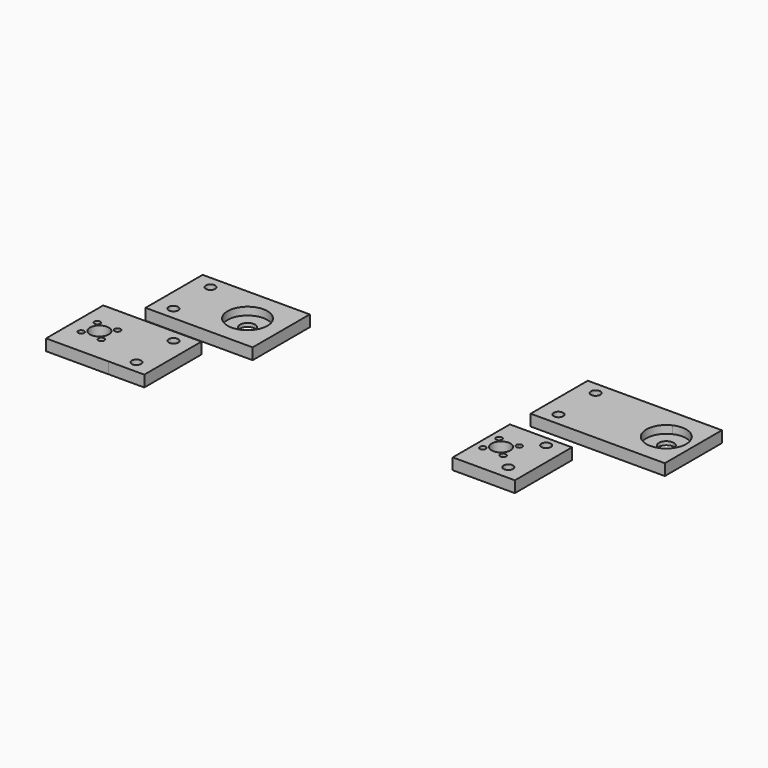
from build123d import *

# Parameters (mm, degrees)
F1_R     = 1.65
F1_R_2   = 5.25
F1_W     = 20
F1_H     = 40
F1_R_3   = 2.65
F2_DEPTH = 6.35
F0_W     = 20
F0_H     = 40
F0_R     = 2.65
F0_W_2   = 40
F0_R_2   = 11.15
F3_DEPTH = 6.35
F0_R_3   = 4.1518260948
F4_DEPTH = 2


# Not quite as in the source:
# - a feature names something its author has since deleted; it is built from what else it names


with BuildPart() as f2:
    # F1 (on Top) → F2 (new body)
    with BuildSketch(Plane.XY):
        Polygon((-72.8019029178, -47.3758022127), (-72.8019029178, -47.3600610539), (-72.8019029178, -7.3600610539), (-102.8019029178, -7.3600610539), (-107.8019029178, -7.3600610539), (-107.8019029178, -47.3758022127), (-102.8956038096, -47.3758022127), align=None)
        with Locations((-99.6128339202, -33.0128356103)):
            Circle(F1_R, mode=Mode.SUBTRACT)
        with Locations((-88.2909719153, -33.0128356103)):
            Circle(F1_R, mode=Mode.SUBTRACT)
        with Locations((-93.9519029178, -27.3600610539)):
            Circle(F1_R_2, mode=Mode.SUBTRACT)
        with Locations((-99.6128339202, -21.7072864974)):
            Circle(F1_R, mode=Mode.SUBTRACT)
        with Locations((-88.2909719153, -21.7072864974)):
            Circle(F1_R, mode=Mode.SUBTRACT)
        with Locations((-62.8019029178, -27.3600610539)):
            Rectangle(F1_W, F1_H)
        with Locations((-62.8019029178, -40.3600610539)):
            Circle(F1_R_3, mode=Mode.SUBTRACT)
        with Locations((-62.8019029178, -14.3600610539)):
            Circle(F1_R_3, mode=Mode.SUBTRACT)
    extrude(amount=F2_DEPTH)


with BuildPart() as f2b:
    # F1 (on Top) → F2, piece 2 (new body)
    with BuildSketch(Plane.XY):
        with BuildLine():
            Line((101.5164678693, -24.2658690363), (116.3195730567, -24.2658690363))
            Line((116.3195730567, -24.2658690363), (116.3195730567, -10.1336148514))
            ThreePointArc((116.3195730567, -10.1336148514), (115.8805040591, -9.0128356103), (116.3195730567, -7.8920563691))
            Line((116.3195730567, -7.8920563691), (116.3195730567, -6.1457387093))
            ThreePointArc((116.3195730567, -6.1457387093), (106.6195730567, -3.3600610539), (116.3195730567, -0.5743833984))
            Line((116.3195730567, -0.5743833984), (116.3195730567, 1.1719342614))
            ThreePointArc((116.3195730567, 1.1719342614), (115.8805040591, 2.2927135026), (116.3195730567, 3.4134927437))
            Line((116.3195730567, 3.4134927437), (116.3195730567, 15.7341309637))
            Line((116.3195730567, 15.7341309637), (101.5164678693, 15.7341309637))
            Line((101.5164678693, 15.7341309637), (101.5164678693, -24.2658690363))
        make_face()
        with Locations((106.2086420543, -9.0128356103)):
            Circle(F1_R, mode=Mode.SUBTRACT)
        with Locations((106.2086420543, 2.2927135026)):
            Circle(F1_R, mode=Mode.SUBTRACT)
        with BuildLine():
            Line((116.3195730567, -24.2658690363), (136.3195730567, -24.2658690363))
            Line((136.3195730567, -24.2658690363), (136.3195730567, 15.7341309637))
            Line((136.3195730567, 15.7341309637), (116.3195730567, 15.7341309637))
            Line((116.3195730567, 15.7341309637), (116.3195730567, 3.4134927437))
            ThreePointArc((116.3195730567, 3.4134927437), (118.1323611211, 3.8290299013), (119.1805040591, 2.2927135026))
            ThreePointArc((119.1805040591, 2.2927135026), (118.1323611211, 0.7563971038), (116.3195730567, 1.1719342614))
            Line((116.3195730567, 1.1719342614), (116.3195730567, -0.5743833984))
            ThreePointArc((116.3195730567, -0.5743833984), (116.9156111065, -1.9109233792), (117.1195730567, -3.3600610539))
            ThreePointArc((117.1195730567, -3.3600610539), (116.9156111065, -4.8091987285), (116.3195730567, -6.1457387093))
            Line((116.3195730567, -6.1457387093), (116.3195730567, -7.8920563691))
            ThreePointArc((116.3195730567, -7.8920563691), (118.1323611211, -7.4765192115), (119.1805040591, -9.0128356103))
            ThreePointArc((119.1805040591, -9.0128356103), (118.1323611211, -10.549152009), (116.3195730567, -10.1336148514))
            Line((116.3195730567, -10.1336148514), (116.3195730567, -24.2658690363))
        make_face()
        with Locations((126.3195730567, -16.3600610539)):
            Circle(F1_R_3, mode=Mode.SUBTRACT)
        with Locations((126.3195730567, 10.1646915369)):
            Circle(F1_R_3, mode=Mode.SUBTRACT)
    extrude(amount=F2_DEPTH)


with BuildPart() as f3:
    # F0 (on Top) → F3 (new body)
    with BuildSketch(Plane.XY):
        with Locations((-81.926522553, 22.4182014516)):
            Rectangle(F0_W, F0_H)
        with Locations((-81.926522553, 9.4182014516)):
            Circle(F0_R, mode=Mode.SUBTRACT)
        with Locations((-81.926522553, 35.4182014516)):
            Circle(F0_R, mode=Mode.SUBTRACT)
        with Locations((-51.926522553, 22.4182014516)):
            Rectangle(F0_W_2, F0_H)
        with Locations((-50.776522553, 22.4182014516)):
            Circle(F0_R_2, mode=Mode.SUBTRACT)
    extrude(amount=F3_DEPTH)

    # F0 (on Top) → F4 (join)
    with BuildSketch(Plane.XY):
        with Locations((-50.776522553, 22.4182014516)):
            Circle(F0_R_2)
        with Locations((-50.776522553, 22.4182014516)):
            Circle(F0_R_3, mode=Mode.SUBTRACT)
    extrude(amount=F4_DEPTH)


with BuildPart() as f3b:
    # F0 (on Top) → F3, piece 2 (new body)
    with BuildSketch(Plane.XY):
        with Locations((112.2669861317, 49.3423603475)):
            Rectangle(F0_W, F0_H)
        with Locations((112.2669861317, 36.3423603475)):
            Circle(F0_R, mode=Mode.SUBTRACT)
        with Locations((112.2669861317, 62.3423603475)):
            Circle(F0_R, mode=Mode.SUBTRACT)
        with BuildLine():
            Line((157.5969861317, 69.3423603475), (122.2669861317, 69.3423603475))
            Line((122.2669861317, 69.3423603475), (122.2669861317, 29.3423603475))
            Line((122.2669861317, 29.3423603475), (157.5969861317, 29.3423603475))
            Line((157.5969861317, 29.3423603475), (157.5969861317, 39.217460348))
            ThreePointArc((157.5969861317, 39.217460348), (151.1169861317, 49.3423603475), (157.5969861317, 59.467260347))
            Line((157.5969861317, 59.467260347), (157.5969861317, 69.3423603475))
        make_face()
        with BuildLine():
            Line((177.4169861317, 69.3423603475), (157.5969861317, 69.3423603475))
            Line((157.5969861317, 69.3423603475), (157.5969861317, 59.467260347))
            ThreePointArc((157.5969861317, 59.467260347), (168.2774769602, 58.7336595122), (173.4169861317, 49.3423603475))
            ThreePointArc((173.4169861317, 49.3423603475), (168.2774769602, 39.9510611829), (157.5969861317, 39.217460348))
            Line((157.5969861317, 39.217460348), (157.5969861317, 29.3423603475))
            Line((157.5969861317, 29.3423603475), (177.4169861317, 29.3423603475))
            Line((177.4169861317, 29.3423603475), (177.4169861317, 69.3423603475))
        make_face()
    extrude(amount=F3_DEPTH)

    # F0 (on Top) → F4, piece 2 (join)
    with BuildSketch(Plane.XY):
        with BuildLine():
            Line((157.5969861317, 39.217460348), (157.5969861317, 59.467260347))
            ThreePointArc((157.5969861317, 59.467260347), (151.1169861317, 49.3423603475), (157.5969861317, 39.217460348))
        make_face()
        with BuildLine():
            ThreePointArc((173.4169861317, 49.3423603475), (168.2774769602, 58.7336595122), (157.5969861317, 59.467260347))
            Line((157.5969861317, 59.467260347), (157.5969861317, 39.217460348))
            ThreePointArc((157.5969861317, 39.217460348), (168.2774769602, 39.9510611829), (173.4169861317, 49.3423603475))
        make_face()
        with Locations((162.2669861317, 49.3423603475)):
            Circle(F0_R_3, mode=Mode.SUBTRACT)
    extrude(amount=F4_DEPTH)


solid = Compound([f2.part, f2b.part, f3.part, f3b.part])
